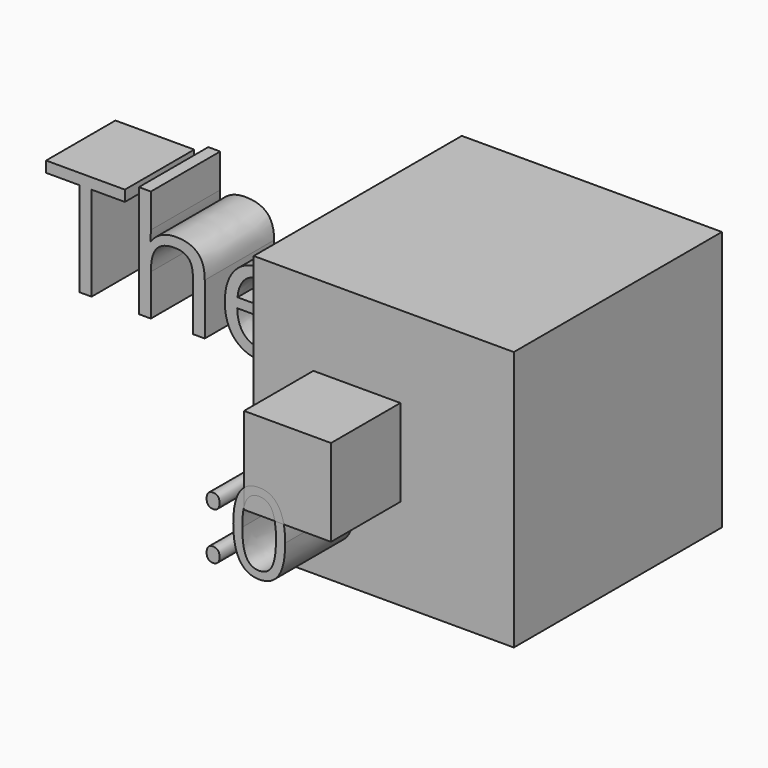
from build123d import *

# Parameters (mm, degrees)
F0_W         = 76.2
F0_H         = 76.2
F1_DEPTH     = 76.2
F2_W         = 25.4814699292
F2_H         = 25.4834927619
F3_DEPTH     = 25.4
F5_TEXT_SIZE = 32.2314082748
F6_DEPTH     = 25.4
F7_TEXT_SIZE = 43.1274684767
F8_DEPTH     = 25.4


# Not quite as in the source:
# - Text() gives the source's letters only with a copy of the font that has no kerning and outlines rounded to 1/6400 em; it was checked with that copy


with BuildPart() as f1:
    # F0 (on Front) → F1 (new body)
    with BuildSketch(Plane.XZ):
        with Locations((38.1, 38.1)):
            Rectangle(F0_W, F0_H)
    extrude(amount=F1_DEPTH)

    # F2 (on face) → F3 (join)
    with BuildSketch(Plane.XZ.offset(76.2)):
        with Locations((30.2292704582, 39.5167823881)):
            Rectangle(F2_W, F2_H)
    extrude(amount=F3_DEPTH)

    # F5 (on face) → F6 (join)
    with BuildSketch(Plane.XZ.offset(76.2)):
        with Locations((4.1413269937, 10.5438232422)):
            Text(':0', F5_TEXT_SIZE, font='Open Sans', text_align=(TextAlign.LEFT, TextAlign.BOTTOM))
    extrude(amount=F6_DEPTH)


with BuildPart() as f8:
    # F7 (on Front) → F8 (new body)
    with BuildSketch(Plane.XZ):
        with Locations((-101.8387228251, 16.3792185485)):
            Text('The', F7_TEXT_SIZE, font='Open Sans', text_align=(TextAlign.LEFT, TextAlign.BOTTOM))
    extrude(amount=F8_DEPTH)


solid = Compound([f1.part, f8.part])
